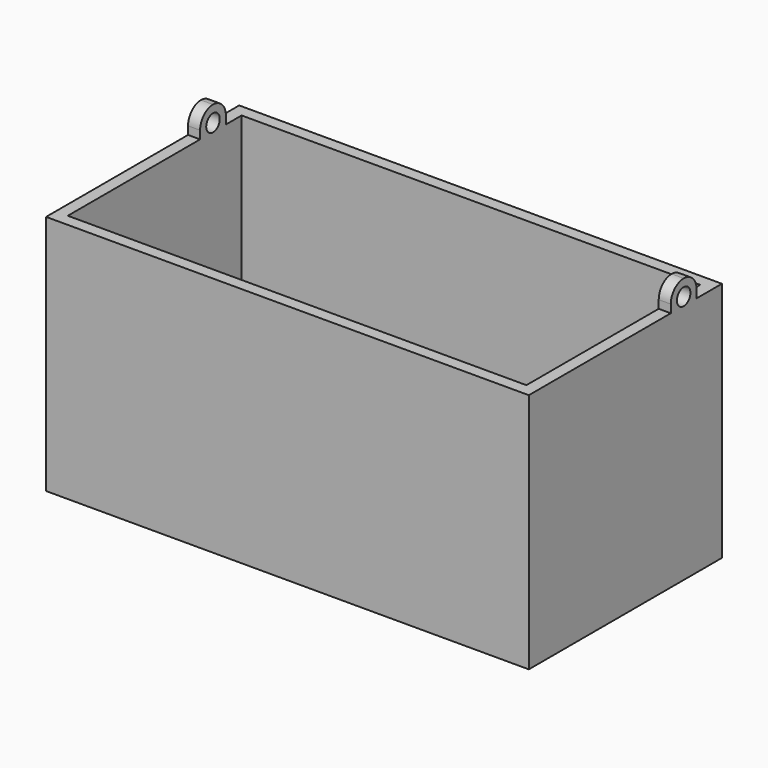
from build123d import *

# Parameters (mm, degrees)
F0_W      = 152.4
F0_H      = 76.2
F1_DEPTH  = 76.2
F2_T      = -3.81
F3_W      = 3.81
F3_H      = 10.16
F4_DEPTH  = 7.62
F5_R      = 2.667
F6_DEPTH  = 152.401
F7_R      = 5.07999
F8_W      = 144.78
F8_H      = 5.08
F9_DEPTH  = 5.08
F11_DEPTH = 144.78


# Not quite as in the source:
# - a fillet or chamfer is up to 0.001 mm smaller than in the source, because OpenCascade refuses the exact size


with BuildPart() as f1:
    # F0 (on Top) → F1 (new body)
    with BuildSketch(Plane.XY):
        Rectangle(F0_W, F0_H)
    extrude(amount=F1_DEPTH)

    # F2
    f2_openings = [f1.faces().sort_by_distance(p)[0] for p in [
        (0, 0, 76.2),
    ]]
    offset(amount=F2_T, openings=f2_openings)

    # F3 (on face) → F4 (join)
    with BuildSketch(Plane.XY.offset(76.2)):
        with Locations((-74.295, 23.0027831805)):
            Rectangle(F3_W, F3_H)
        with Locations((74.295, 23.0027831805)):
            Rectangle(F3_W, F3_H)
    extrude(amount=F4_DEPTH)

    # F5 (on face) → F6 (cut, through all)
    with BuildSketch(Plane.YZ.offset(76.2)):
        with Locations((23.0027831805, 78.74)):
            Circle(F5_R)
    extrude(amount=-F6_DEPTH, mode=Mode.SUBTRACT)

    # F7 (radius 5.08 in the source; OpenCascade refuses exactly that, so slightly less here)
    f7_edges = [f1.edges().sort_by_distance(p)[0] for p in [
        (74.295, 17.922783, 83.82),
        (74.295, 28.082783, 83.82),
        (-74.295, 28.082783, 83.82),
        (-74.295, 17.922783, 83.82),
    ]]
    fillet(f7_edges, radius=F7_R)

    # F8 (on face) → F9 (join)
    with BuildSketch(Plane(origin=(0, -34.29, 0), x_dir=(-1, 0, 0), z_dir=(0, 1, 0))):
        with Locations((0, 68.58)):
            Rectangle(F8_W, F8_H)
    extrude(amount=F9_DEPTH)

    # F10 (on face) → F11 (join)
    with BuildSketch(Plane.YZ.offset(-72.39)):
        Polygon((-34.29, 60.96), (-29.21, 66.04), (-34.29, 66.04), align=None)
    extrude(amount=F11_DEPTH)


solid = f1.part
